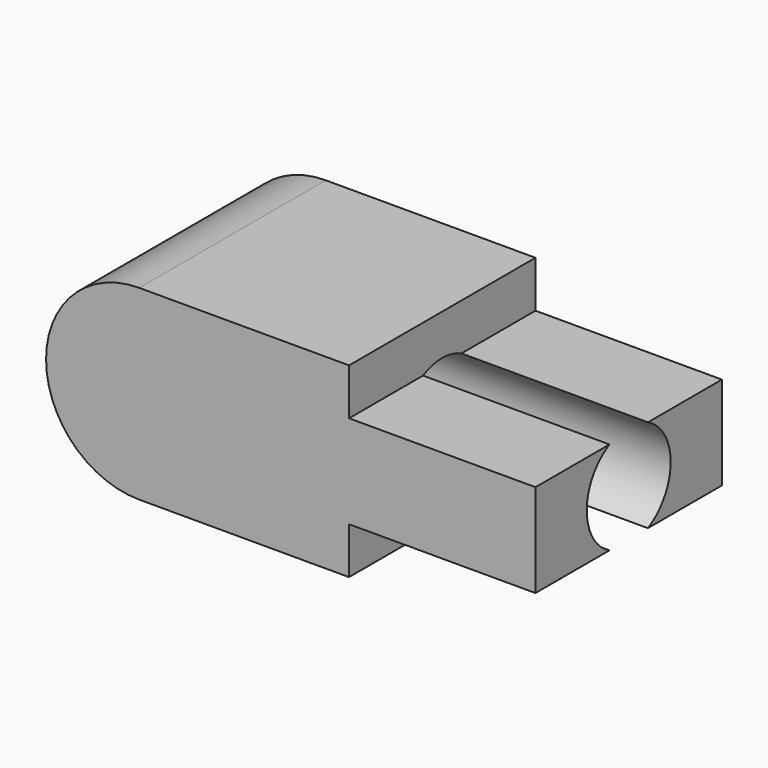
from build123d import *
from build123d import SkipClean  # not in build123d's __all__

# Parameters (mm, degrees)
F0_W     = 1016
F0_H     = 812.8
F0_R     = 228.6
F1_DEPTH = 2133.6
F2_W     = 812.8
F2_H     = 203.2
F3_DEPTH = 1016.001


with BuildPart() as f1:
    # F0 (on Right) → F1 (new body)
    with BuildSketch(Plane.YZ):
        with Locations((432.4176223874, 331.1518777847)):
            Rectangle(F0_W, F0_H)
        with Locations((432.4176223874, 331.1518777847)):
            Circle(F0_R, mode=Mode.SUBTRACT)
    extrude(amount=F1_DEPTH)

    # F2 (on face) → F3 (cut, through all)
    with BuildSketch(Plane.XZ.offset(75.5823776126)):
        with BuildLine():
            Line((0, 737.5518777847), (0, 331.1518777847))
            ThreePointArc((0, 331.1518777847), (119.0318041258, 618.5200736589), (406.4, 737.5518777847))
            Line((406.4, 737.5518777847), (0, 737.5518777847))
        make_face()
        with BuildLine():
            Line((0, 331.1518777847), (0, -75.2481222153))
            Line((0, -75.2481222153), (406.4, -75.2481222153))
            ThreePointArc((406.4, -75.2481222153), (119.0318041258, 43.7836819105), (0, 331.1518777847))
        make_face()
        with Locations((1727.2, 26.3518777847)):
            Rectangle(F2_W, F2_H)
        with Locations((1727.2, 635.9518777847)):
            Rectangle(F2_W, F2_H)
    with SkipClean():  # cleaning this boolean's faces spoils the solid; the shape is the same uncleaned
        extrude(amount=-F3_DEPTH, mode=Mode.SUBTRACT)


solid = f1.part
